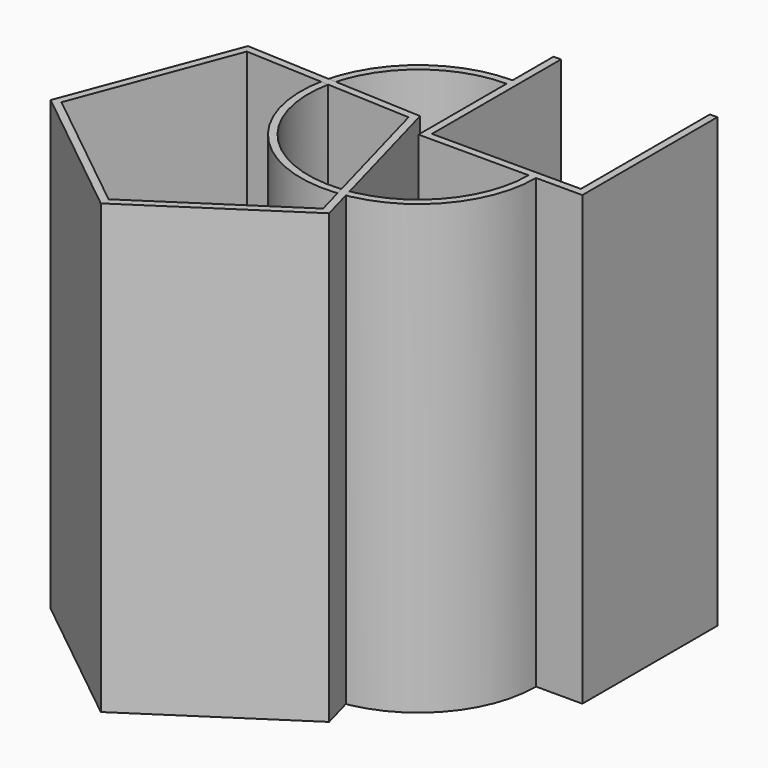
from build123d import *

# Parameters (mm, degrees)
F0_R         = 39.3858974646
F1_DEPTH     = 150
F2_T         = -2.5
F3_W         = 54.8863634467
F3_H         = 56.5410479903
F4_DEPTH     = 150
F5_T         = 2.5
F5_T3_DEPTH  = 155
F5_T5_DEPTH  = 152.5
F5_T7_DEPTH  = 41.8858974646
F5_T9_DEPTH  = 41.8858974646
F5_T12_ANGLE = 270.000000001
F7_DEPTH     = 150
F8_T         = -2.5


# Not quite as in the source:
# - a shell that OpenCascade refuses in one call is made with other operations: the cavity is built on its own and cut out


with BuildPart() as f1:
    # F0 (on Top) → F1 (new body)
    with BuildSketch(Plane.XY):
        Circle(F0_R)
    extrude(amount=F1_DEPTH)

    # F2
    f2_openings = [f1.faces().sort_by_distance(p)[0] for p in [
        (0, 0, 150),
    ]]
    offset(amount=F2_T, openings=f2_openings)

    # F3 (on Top) → F4 (join)
    with BuildSketch(Plane.XY):
        with Locations((27.4431817234, 28.2705239952)):
            Rectangle(F3_W, F3_H)
    extrude(amount=F4_DEPTH)

    # F5: shell of thickness 2.5, made by hand


with BuildPart() as f5_core1:
    # F5_t2: copy of F1
    add(f1.part)

    # the walls: a layer under each face that stays
    f5_faces = [f5_core1.faces().sort_by_distance(p)[0] for p in [
        (7.7502329911, 8.5775752629, 0),
        (-27.8500351803, -27.8500351803, 75),
        (54.8863634467, 28.2705239952, 75),
        (47.1361304556, 0, 75),
        (0, 47.9634727274, 75),
        (-26.0822682274, -26.0822682273, 76.25),
        (18.4429487323, 0, 76.25),
        (0, 18.4429487323, 76.25),
        (-24.5905983097, -24.5905983097, 2.5),
    ]]
    thicken(f5_faces, amount=-F5_T, mode=Mode.SUBTRACT)

    # F5_s4 → F5_t3 (cut)
    with BuildSketch(Plane.XY.offset(-2.5)):
        Polygon((39.4108974646, -0.025), (36.8858974646, 0), (36.8858974646, 2.5), (39.3858974646, 2.5), align=None)
        Polygon((-0.025, 39.4108974646), (0, 36.8858974646), (2.5, 36.8858974646), (2.5, 39.3858974646), align=None)
    extrude(amount=F5_T3_DEPTH, mode=Mode.SUBTRACT)

    # F5_s6 → F5_t5 (cut)
    with BuildSketch(Plane.XY):
        Polygon((36.8608974646, -0.025), (39.3858974646, 0), (39.3858974646, 2.5), (36.8858974646, 2.5), align=None)
        Polygon((-0.025, 36.8608974646), (0, 39.3858974646), (2.5, 39.3858974646), (2.5, 36.8858974646), align=None)
    extrude(amount=F5_T5_DEPTH, mode=Mode.SUBTRACT)

    # F5_s8 → F5_t7 (cut)
    with BuildSketch(Plane.YZ.offset(-2.5)):
        Polygon((-0.025, 2.525), (2.5, 2.5), (2.5, 0), (0, 0), align=None)
    extrude(amount=F5_T7_DEPTH, mode=Mode.SUBTRACT)

    # F5_s10 → F5_t9 (cut)
    with BuildSketch(Plane.XZ.offset(-39.3858974646)):
        Polygon((-0.025, 2.525), (2.5, 2.5), (2.5, 0), (0, 0), align=None)
    extrude(amount=F5_T9_DEPTH, mode=Mode.SUBTRACT)

    # F5_s11 → F5_t12 (revolve, cut)
    with BuildSketch(Plane.XZ):
        Polygon((36.8608974646, 2.525), (39.3858974646, 2.5), (39.3858974646, 0), (36.8858974646, 0), align=None)
    revolve(axis=Axis((0, 0, 2.5), (0, 0, -1)), revolution_arc=F5_T12_ANGLE, mode=Mode.SUBTRACT)


with BuildPart() as f1_1:
    add(f1.part)

    # what is left inside the walls is the cavity
    f5_cavity = [f5_core1.part.solids().sort_by_distance(p)[0] for p in [
        (52.361363, 29.520524, 100.833333),
    ]]
    add(f5_cavity, mode=Mode.SUBTRACT)


with BuildPart() as f7:
    # F6 (on Top) → F7 (new body)
    with BuildSketch(Plane.XY):
        Polygon((-87.3583794889, -44.8397668156), (-40.5461250487, -82.3494074789), (9.5934452951, -49.4194242689), (-6.2308504914, 8.4420652671), (-66.1503734792, 11.2724492301), align=None)
    extrude(amount=F7_DEPTH)

    # F8
    f8_openings = [f7.faces().sort_by_distance(p)[0] for p in [
        (-38.138457, -31.378817, 150),
    ]]
    offset(amount=F8_T, openings=f8_openings)


solid = Compound([f1_1.part, f7.part])
